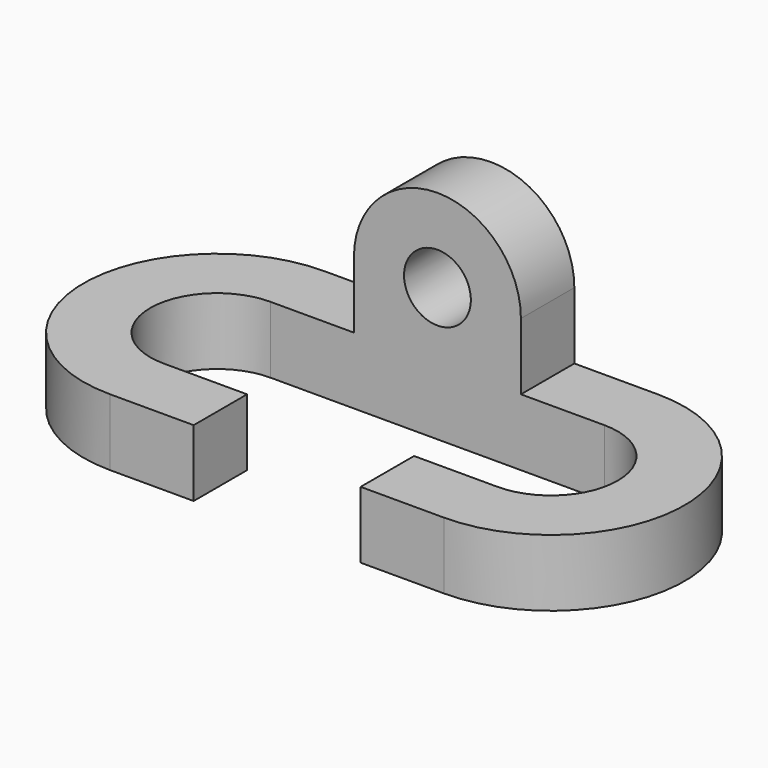
from build123d import *

# Parameters (mm, degrees)
F1_DEPTH = 12.7
F3_R     = 6.35
F4_DEPTH = 12.7


# Not quite as in the source:
# - a feature names something its author has since deleted; it is built from what else it names


with BuildPart() as f1:
    # F0 (on Top) → F1 (new body)
    with BuildSketch(Plane.XY):
        with BuildLine():
            Line((-15.875, -25.4), (0, -25.4))
            ThreePointArc((0, -25.4), (25.4, 0), (0, 25.4))
            Line((0, 25.4), (-31.75, 25.4))
            Line((-31.75, 25.4), (-31.75, 12.7))
            Line((-31.75, 12.7), (0, 12.7))
            ThreePointArc((0, 12.7), (12.7, 0), (0, -12.7))
            Line((0, -12.7), (-15.875, -12.70000043))
            Line((-15.875, -12.70000043), (-15.875, -25.4))
        make_face()
    extrude(amount=F1_DEPTH)

    # F2: F1 across face


with BuildPart() as f1_1:
    add(f1.part)
    add(f1.part.mirror(Plane(origin=(-31.75, 19.05, 6.35), x_dir=(0, -1, 0), z_dir=(-1, 0, 0))))

    # F3 (on face) → F4 (join, through all)
    with BuildSketch(Plane(origin=(0, 25.4, 0), x_dir=(-1, 0, 0), z_dir=(0, 1, 0))):
        with BuildLine():
            Line((47.625, 12.7), (47.625, 25.4))
            ThreePointArc((47.625, 25.4), (31.75, 41.275), (15.875, 25.4))
            Line((15.875, 25.4), (15.875, 12.7))
            Line((15.875, 12.7), (47.625, 12.7))
        make_face()
        with Locations((31.75, 25.4)):
            Circle(F3_R, mode=Mode.SUBTRACT)
    extrude(amount=-F4_DEPTH)


solid = f1_1.part
